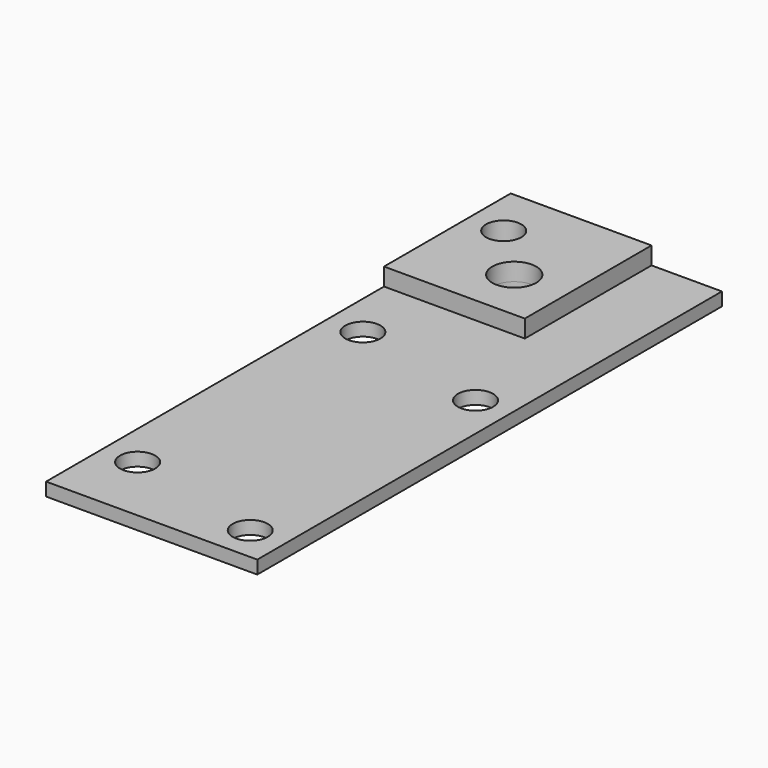
from build123d import *

# Parameters (mm, degrees)
F0_W     = 101.6
F0_H     = 114.3
F0_R     = 15.875
F0_R_2   = 12.7
F1_DEPTH = 12.7
F2_W     = 101.6
F2_H     = 114.3
F2_R     = 12.7
F2_R_2   = 15.875
F3_DEPTH = 9.525


with BuildPart() as f1:
    # F0 (on Top) → F1 (new body)
    with BuildSketch(Plane.XY):
        with Locations((-12.7, 19.05)):
            Rectangle(F0_W, F0_H)
        Circle(F0_R, mode=Mode.SUBTRACT)
        with Locations((-38.1, 38.1)):
            Circle(F0_R_2, mode=Mode.SUBTRACT)
    extrude(amount=F1_DEPTH)


with BuildPart() as f3:
    # F2 (on face) → F3 (new body)
    with BuildSketch(Plane(origin=(0, 0, 0), x_dir=(1, 0, 0), z_dir=(0, 0, -1))):
        with Locations((-12.7, -19.05)):
            Rectangle(F2_W, F2_H)
        with Locations((-38.1, -38.1)):
            Circle(F2_R, mode=Mode.SUBTRACT)
        Circle(F2_R_2, mode=Mode.SUBTRACT)
        Polygon((38.1, 38.1), (38.1, -76.2), (88.9, -76.2), (88.9, 342.9), (-63.5, 342.9), (-63.5, 38.1), align=None)
        with Locations((-38.1, 88.9)):
            Circle(F2_R, mode=Mode.SUBTRACT)
        with Locations((63.5, 114.3)):
            Circle(F2_R, mode=Mode.SUBTRACT)
        with Locations((-38.1, 292.1)):
            Circle(F2_R, mode=Mode.SUBTRACT)
        with Locations((63.5, 317.5)):
            Circle(F2_R, mode=Mode.SUBTRACT)
    extrude(amount=F3_DEPTH)


solid = Compound([f1.part, f3.part])
